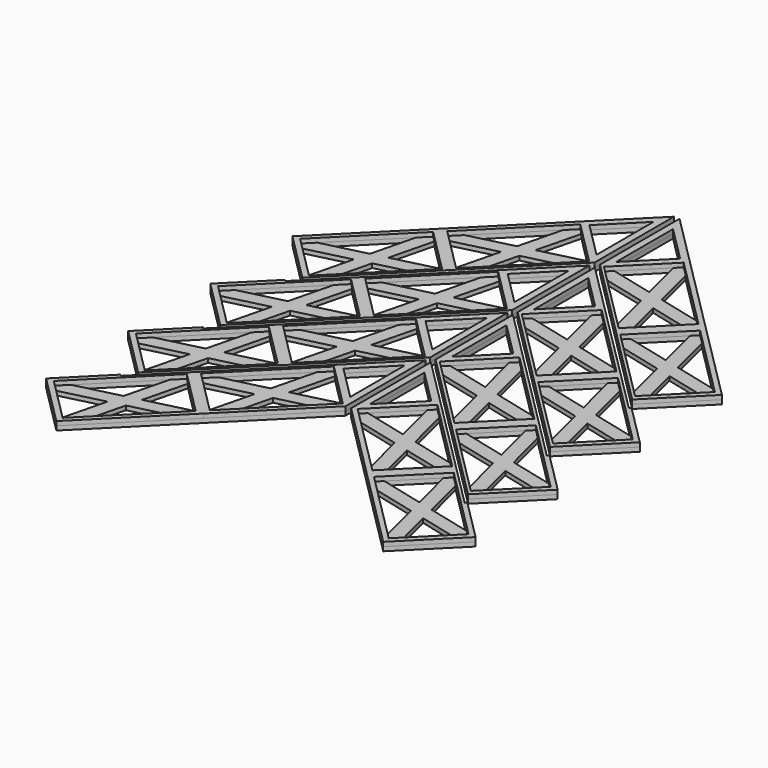
from build123d import *

# Parameters (mm, degrees)
F1_DEPTH = 3
F3_DEPTH = 3
F5_DEPTH = 6
F7_DEPTH = 6


# Not quite as in the source:
# - a feature names something its author has since deleted; it is built from what else it names


with BuildPart() as f1:
    # F0 (on Top) → F1 (new body)
    with BuildSketch(Plane.XY):
        Polygon((-2, -61.6396103068), (-2, -2), (-31.8198051534, -31.8198051534), align=None)
        Polygon((-2, -61.6396103068), (-31.8198051534, -31.8198051534), (-36.8198067184, -36.8198067184), (-2, -71.6396104532), align=None)
        Polygon((-2, -71.6396104532), (-36.8198067184, -36.8198067184), (-95.4594154602, -95.4594154602), (-59.7206892891, -131.1346304254), (-2, -73.3111832249), align=None)
        Polygon((-90.1561136766, -95.1561166906), (-37.1231070285, -42.1231061606), (-5.3033007106, -73.9429101495), (-58.3363073586, -126.9759206794), align=None, mode=Mode.SUBTRACT)
        Polygon((-59.7206892891, -131.1346304254), (-95.4594154602, -95.4594154602), (-154.0990202856, -154.0990288702), (-118.3398738044, -189.8581724084), align=None)
        Polygon((-148.7957204896, -153.795727796), (-95.7627138416, -100.762717266), (-63.9429075236, -132.5825212548), (-116.9759141717, -185.6155317848), align=None, mode=Mode.SUBTRACT)
    extrude(amount=F1_DEPTH)


with BuildPart() as f1b:
    # F0 (on Top) → F1, piece 2 (new body)
    with BuildSketch(Plane.XY):
        Polygon((-123.2896154271, -346.3297840758), (-124.3502800956, -345.2691194021), (-154.0990289767, -375.0178411307), (-117.2792322747, -411.8376540035), (-58.6396110618, -353.198051557), (-94.398746738, -317.4389106458), align=None)
        Polygon((-148.7957294692, -374.7145407415), (-95.7627092344, -321.6815437982), (-63.9429110685, -353.501355939), (-116.9759313032, -406.5343528823), align=None, mode=Mode.SUBTRACT)
        Polygon((-2, -292.5584394851), (-2, -282.558438898), (-30.7591427167, -253.7992961813), (-35.7591450711, -258.7992993562), align=None)
        Polygon((-2, -282.558438898), (-2, -225.0401487453), (-30.7591427167, -253.7992961813), align=None)
        Polygon((-2, -296.5584389525), (-2, -292.5584394851), (-35.7591450711, -258.7992993562), (-94.398746738, -317.4389106458), (-58.6396110618, -353.198051557), align=None)
        Polygon((-90.1561133859, -316.0749487705), (-37.1231086789, -263.0419362996), (-5.3033011963, -294.8617391239), (-58.3363059034, -347.8947515948), align=None, mode=Mode.SUBTRACT)
    extrude(amount=F1_DEPTH)


with BuildPart() as f1c:
    # F0 (on Top) → F1, piece 3 (new body)
    with BuildSketch(Plane.XY):
        Polygon((-123.2896235896, -272.6901718374), (-124.3502835323, -271.62951205), (-154.0990146791, -301.3782501328), (-118.3398697839, -337.1373952008), (-59.7002649834, -278.4977817547), (-94.3987529307, -243.7992988871), align=None)
        Polygon((-116.9759095702, -332.8947529571), (-148.7957170528, -301.0749501328), (-95.7627123456, -248.041937662), (-63.9429048631, -279.8617404862), align=None, mode=Mode.SUBTRACT)
        Polygon((-2, -218.9188283053), (-2, -208.9188285912), (-30.7591438411, -180.1596847501), (-35.7591485237, -185.1596898292), align=None)
        Polygon((-2, -208.9188285912), (-2, -151.400538628), (-30.7591438411, -180.1596847501), align=None)
        Polygon((-2, -220.7975082642), (-2, -218.9188283053), (-35.7591485237, -185.1596898292), (-94.3987529307, -243.7992988871), (-59.7002649834, -278.4977817547), align=None)
        Polygon((-90.1561143554, -242.435338851), (-37.1231096484, -189.4023263801), (-5.3033021659, -221.2221292043), (-58.336306873, -274.2551416752), align=None, mode=Mode.SUBTRACT)
    extrude(amount=F1_DEPTH)


with BuildPart() as f1d:
    # F0 (on Top) → F1, piece 4 (new body)
    with BuildSketch(Plane.XY):
        Polygon((-2, -135.3278050504), (-2, -77.9680376814), (-30.6798418058, -106.5989096283), align=None)
        Polygon((-2, -145.3363573492), (-2, -135.3278050504), (-30.6798418058, -106.5989096283), (-35.6841106479, -111.5946338508), align=None)
        Polygon((-123.2896209509, -199.050560711), (-124.3502811379, -197.9899006113), (-154.099019893, -227.7386418146), (-118.3398762823, -263.4977828078), (-59.7002682444, -204.8581704429), (-94.374065836, -170.1843779274), align=None)
        Polygon((-95.7627149147, -174.4023288289), (-63.9429093731, -206.2221297122), (-116.9759140802, -259.2551421831), (-148.7957196218, -227.4353412998), align=None, mode=Mode.SUBTRACT)
        Polygon((-2, -147.1578979409), (-2, -145.3363573492), (-35.6841106479, -111.5946338508), (-94.374065836, -170.1843779274), (-59.7002682444, -204.8581704429), align=None)
        Polygon((-37.1231038315, -115.7627173353), (-5.3033006191, -147.5825205477), (-58.336309208, -200.6155291367), (-90.1561124205, -168.7957259243), align=None, mode=Mode.SUBTRACT)
    extrude(amount=F1_DEPTH)


with BuildPart() as f1e:
    # F0 (on Top) → F1, piece 5 (new body)
    with BuildSketch(Plane.XY):
        Polygon((31.8198051534, -31.8198051534), (2, -2), (2, -61.6396103068), align=None)
        Polygon((31.8198051534, -31.8198051534), (2, -61.6396103068), (2, -71.6396104532), (36.8198067184, -36.8198067184), align=None)
        Polygon((36.8198067184, -36.8198067184), (2, -71.6396104532), (2, -73.3111832249), (59.7206892891, -131.1346304254), (95.4594154602, -95.4594154602), align=None)
        Polygon((37.1231070285, -42.1231061606), (90.1561136766, -95.1561166906), (58.3363073586, -126.9759206794), (5.3033007106, -73.9429101495), align=None, mode=Mode.SUBTRACT)
        Polygon((154.0990202856, -154.0990288702), (95.4594154602, -95.4594154602), (59.7206892891, -131.1346304254), (118.3398738044, -189.8581724084), align=None)
        Polygon((63.9429075236, -132.5825212548), (95.7627138416, -100.762717266), (148.7957204896, -153.795727796), (116.9759141717, -185.6155317848), align=None, mode=Mode.SUBTRACT)
    extrude(amount=F1_DEPTH)


with BuildPart() as f1f:
    # F0 (on Top) → F1, piece 6 (new body)
    with BuildSketch(Plane.XY):
        Polygon((30.6798418058, -106.5989096283), (2, -77.9680376814), (2, -135.3278050504), align=None)
        Polygon((30.6798418058, -106.5989096283), (2, -135.3278050504), (2, -145.3363573492), (35.6841106479, -111.5946338508), align=None)
        Polygon((35.6841106479, -111.5946338508), (2, -145.3363573492), (2, -147.1578979409), (59.7002682444, -204.8581704429), (94.374065836, -170.1843779274), align=None)
        Polygon((58.336309208, -200.6155291367), (5.3033006191, -147.5825205477), (37.1231038315, -115.7627173353), (90.1561124205, -168.7957259243), align=None, mode=Mode.SUBTRACT)
        Polygon((123.2896209509, -199.050560711), (94.374065836, -170.1843779274), (59.7002682444, -204.8581704429), (118.3398762823, -263.4977828078), (154.099019893, -227.7386418146), (124.3502811379, -197.9899006113), align=None)
        Polygon((63.9429093731, -206.2221297122), (95.7627149147, -174.4023288289), (148.7957196217, -227.4353412998), (116.9759140802, -259.2551421831), align=None, mode=Mode.SUBTRACT)
    extrude(amount=F1_DEPTH)


with BuildPart() as f1g:
    # F0 (on Top) → F1, piece 7 (new body)
    with BuildSketch(Plane.XY):
        Polygon((30.7591438411, -180.1596847501), (2, -151.400538628), (2, -208.9188285912), align=None)
        Polygon((30.7591438411, -180.1596847501), (2, -208.9188285912), (2, -218.9188283053), (35.7591485237, -185.1596898292), align=None)
        Polygon((35.7591485237, -185.1596898292), (2, -218.9188283053), (2, -220.7975082642), (59.7002649834, -278.4977817547), (94.3987529307, -243.7992988871), align=None)
        Polygon((5.3033021659, -221.2221292043), (37.1231096484, -189.4023263801), (90.1561143554, -242.435338851), (58.336306873, -274.2551416752), align=None, mode=Mode.SUBTRACT)
        Polygon((123.2896235896, -272.6901718374), (94.3987529307, -243.7992988871), (59.7002649834, -278.4977817547), (118.3398697839, -337.1373952008), (154.0990146791, -301.3782501328), (124.3502835323, -271.62951205), align=None)
        Polygon((116.9759095702, -332.8947529571), (63.9429048631, -279.8617404862), (95.7627123456, -248.041937662), (148.7957170528, -301.0749501328), align=None, mode=Mode.SUBTRACT)
    extrude(amount=F1_DEPTH)


with BuildPart() as f1h:
    # F0 (on Top) → F1, piece 8 (new body)
    with BuildSketch(Plane.XY):
        Polygon((30.7591427167, -253.7992961813), (2, -225.0401487453), (2, -282.558438898), align=None)
        Polygon((30.7591427167, -253.7992961813), (2, -282.558438898), (2, -292.5584394851), (35.7591450711, -258.7992993562), align=None)
        Polygon((35.7591450711, -258.7992993562), (2, -292.5584394851), (2, -296.5584389525), (58.6396110618, -353.198051557), (94.398746738, -317.4389106458), align=None)
        Polygon((5.3033011963, -294.8617391239), (37.1231086789, -263.0419362996), (90.1561133859, -316.0749487705), (58.3363059034, -347.8947515948), align=None, mode=Mode.SUBTRACT)
        Polygon((123.2896154271, -346.3297840758), (94.398746738, -317.4389106458), (58.6396110618, -353.198051557), (117.2792322747, -411.8376540035), (154.0990289767, -375.0178411307), (124.3502800956, -345.2691194021), align=None)
        Polygon((95.7627092344, -321.6815437982), (148.7957294692, -374.7145407415), (116.9759313032, -406.5343528823), (63.9429110685, -353.501355939), align=None, mode=Mode.SUBTRACT)
    extrude(amount=F1_DEPTH)


with BuildPart() as f3:
    # F2 (on face) → F3 (new body)
    with BuildSketch(Plane(origin=(0, 0, 0), x_dir=(1, 0, 0), z_dir=(0, 0, -1))):
        Polygon((2, 73.3111832249), (2, 2), (154.0990202856, 154.0990288702), (118.3398738044, 189.8581724084), align=None)
        Polygon((33.000001252, 46.2462116354), (9.4264064871, 69.8198046747), (40.8578647357, 77.6776704592), align=None, mode=Mode.SUBTRACT)
        Polygon((12.1751431684, 80.8147531103), (51.4644649007, 120.1040777185), (43.606601417, 88.6726188947), align=None, mode=Mode.SUBTRACT)
        Polygon((83.2842712187, 88.2842737297), (43.9949494864, 48.9949491215), (51.8528129701, 80.4264079453), align=None, mode=Mode.SUBTRACT)
        Polygon((62.4594131351, 122.8528152047), (86.0330079, 99.2792221653), (54.6015496514, 91.4213563809), align=None, mode=Mode.SUBTRACT)
        Polygon((91.6396080651, 104.8858227407), (68.0660133001, 128.4594157801), (99.4974715488, 136.3172815645), align=None, mode=Mode.SUBTRACT)
        Polygon((141.9238780318, 146.9238848351), (102.6345562995, 107.6345602269), (110.4924197831, 139.0660190507), align=None, mode=Mode.SUBTRACT)
        Polygon((70.8147499815, 139.4543642157), (110.1040717138, 178.7436888239), (102.2462082301, 147.3122300001), align=None, mode=Mode.SUBTRACT)
        Polygon((121.0990199482, 181.4924263101), (144.6726147131, 157.9188332707), (113.2411564645, 150.0609674863), align=None, mode=Mode.SUBTRACT)
    extrude(amount=F3_DEPTH)


with BuildPart() as f3b:
    # F2 (on face) → F3, piece 2 (new body)
    with BuildSketch(Plane(origin=(0, 0, 0), x_dir=(1, 0, 0), z_dir=(0, 0, -1))):
        Polygon((2, 147.1578979409), (2, 77.9680376814), (123.2896209509, 199.050560711), (124.3502811379, 197.9899006113), (154.099019893, 227.7386418146), (118.3398762823, 263.4977828078), align=None)
        Polygon((32.9999982725, 119.8858228944), (9.4264061781, 143.4594149887), (40.8578635022, 151.3172802184), align=None, mode=Mode.SUBTRACT)
        Polygon((83.2842694029, 161.9238829067), (43.9949468491, 122.6345603529), (51.8528120788, 154.066017677), align=None, mode=Mode.SUBTRACT)
        Polygon((12.1751436366, 154.4543635653), (51.4644661905, 193.7436861192), (43.6066009607, 162.3122287951), align=None, mode=Mode.SUBTRACT)
        Polygon((62.4594147671, 196.4924235777), (86.0330068614, 172.9188314833), (54.6015495373, 165.0609662536), align=None, mode=Mode.SUBTRACT)
        Polygon((91.6396090538, 178.5254340861), (68.0660152339, 202.0990244549), (99.4974719828, 209.9568919854), align=None, mode=Mode.SUBTRACT)
        Polygon((141.9238771072, 220.5634977792), (102.6345574293, 181.2741723495), (110.4924203583, 212.7056302487), align=None, mode=Mode.SUBTRACT)
        Polygon((70.8147518877, 213.0939732327), (110.1040715656, 252.3832986625), (102.2462086366, 220.9518407632), align=None, mode=Mode.SUBTRACT)
        Polygon((121.099019941, 255.1320369258), (144.6726137609, 231.558446557), (113.241157012, 223.7005790266), align=None, mode=Mode.SUBTRACT)
    extrude(amount=F3_DEPTH)


with BuildPart() as f3c:
    # F2 (on face) → F3, piece 3 (new body)
    with BuildSketch(Plane(origin=(0, 0, 0), x_dir=(1, 0, 0), z_dir=(0, 0, -1))):
        Polygon((154.0990146791, 301.3782501328), (118.3398697839, 337.1373952008), (2, 220.7975082642), (2, 151.400538628), (123.2896235896, 272.6901718374), (124.3502835323, 271.62951205), align=None)
        Polygon((40.8578660543, 224.9568908153), (33.000003721, 193.5254317039), (9.4264080933, 217.0990238805), align=None, mode=Mode.SUBTRACT)
        Polygon((43.6066023333, 235.9518393515), (12.1751443722, 228.0939724167), (51.4644646666, 267.3832984629), align=None, mode=Mode.SUBTRACT)
        Polygon((51.8528141881, 227.7056287039), (83.2842721491, 235.5634956387), (43.9949518547, 196.2741695924), align=None, mode=Mode.SUBTRACT)
        Polygon((54.601550467, 238.7005772401), (62.4594128004, 270.1320363514), (86.033008428, 246.5584441749), align=None, mode=Mode.SUBTRACT)
        Polygon((99.4974687516, 283.5965020972), (91.6396064182, 252.1650429858), (68.0660107905, 275.7386351624), align=None, mode=Mode.SUBTRACT)
        Polygon((102.2462050305, 294.5914506333), (70.8147470695, 286.7335836986), (110.1040673639, 326.0229097447), align=None, mode=Mode.SUBTRACT)
        Polygon((110.4924168853, 286.3452399857), (141.9238748464, 294.2031069205), (102.634554552, 254.9137808744), align=None, mode=Mode.SUBTRACT)
        Polygon((113.2411531643, 297.3401885218), (121.0990154976, 328.7716476333), (144.6726111254, 305.1980554566), align=None, mode=Mode.SUBTRACT)
    extrude(amount=F3_DEPTH)


with BuildPart() as f3d:
    # F2 (on face) → F3, piece 4 (new body)
    with BuildSketch(Plane(origin=(0, 0, 0), x_dir=(1, 0, 0), z_dir=(0, 0, -1))):
        Polygon((2, 296.5584389525), (2, 225.0401487453), (123.2896154271, 346.3297840758), (124.3502800956, 345.2691194021), (154.0990289767, 375.0178411307), (117.2792322747, 411.8376540035), align=None)
        Polygon((33.0000027514, 267.1650416234), (9.4264071237, 290.7386338), (40.8578649974, 298.5965006474), align=None, mode=Mode.SUBTRACT)
        Polygon((83.2842709742, 309.2031053528), (43.9949506799, 269.9137793066), (51.8528131006, 301.3452385054), align=None, mode=Mode.SUBTRACT)
        Polygon((12.1751433489, 301.7335823953), (51.4644634917, 341.022908177), (43.6066012804, 309.5914492918), align=None, mode=Mode.SUBTRACT)
        Polygon((62.4594118308, 343.7716462709), (86.0330074585, 320.1980540943), (54.6015494358, 312.340187175), align=None, mode=Mode.SUBTRACT)
        Polygon((99.4974761378, 357.2361072273), (91.6396045142, 325.8046503292), (68.0660157887, 349.378249408), align=None, mode=Mode.SUBTRACT)
        Polygon((110.4924249682, 359.9848418925), (141.9238854561, 367.8426997465), (102.6345533938, 328.5533850524), align=None, mode=Mode.SUBTRACT)
        Polygon((102.2462157015, 368.2310551291), (70.8147554922, 360.3731973448), (110.1040872902, 399.6625118873), align=None, mode=Mode.SUBTRACT)
        Polygon((113.241164519, 370.979789791), (121.0990360234, 402.4112463513), (144.6726245025, 378.8376475189), align=None, mode=Mode.SUBTRACT)
    extrude(amount=F3_DEPTH)


with BuildPart() as f3e:
    # F2 (on face) → F3, piece 5 (new body)
    with BuildSketch(Plane(origin=(0, 0, 0), x_dir=(1, 0, 0), z_dir=(0, 0, -1))):
        Polygon((-2, 77.9680376814), (-2, 147.1578979409), (-118.3398762823, 263.4977828078), (-154.099019893, 227.7386418146), (-124.3502811379, 197.9899006113), (-123.2896209509, 199.050560711), align=None)
        Polygon((-141.9238771072, 220.5634977792), (-110.4924203583, 212.7056302487), (-102.6345574293, 181.2741723495), align=None, mode=Mode.SUBTRACT)
        Polygon((-99.4974719828, 209.9568919854), (-68.0660152339, 202.0990244549), (-91.6396090538, 178.5254340861), align=None, mode=Mode.SUBTRACT)
        Polygon((-43.9949468491, 122.6345603529), (-83.2842694029, 161.9238829067), (-51.8528120788, 154.066017677), align=None, mode=Mode.SUBTRACT)
        Polygon((-40.8578635022, 151.3172802184), (-9.4264061781, 143.4594149887), (-32.9999982725, 119.8858228944), align=None, mode=Mode.SUBTRACT)
        Polygon((-54.6015495373, 165.0609662536), (-86.0330068614, 172.9188314833), (-62.4594147671, 196.4924235777), align=None, mode=Mode.SUBTRACT)
        Polygon((-12.1751436366, 154.4543635653), (-43.6066009607, 162.3122287951), (-51.4644661905, 193.7436861192), align=None, mode=Mode.SUBTRACT)
        Polygon((-113.241157012, 223.7005790266), (-144.6726137609, 231.558446557), (-121.099019941, 255.1320369258), align=None, mode=Mode.SUBTRACT)
        Polygon((-70.8147518877, 213.0939732327), (-102.2462086366, 220.9518407632), (-110.1040715656, 252.3832986625), align=None, mode=Mode.SUBTRACT)
    extrude(amount=F3_DEPTH)


with BuildPart() as f3f:
    # F2 (on face) → F3, piece 6 (new body)
    with BuildSketch(Plane(origin=(0, 0, 0), x_dir=(1, 0, 0), z_dir=(0, 0, -1))):
        Polygon((-2, 2), (-2, 73.3111832249), (-118.3398738044, 189.8581724084), (-154.0990202856, 154.0990288702), align=None)
        Polygon((-83.2842712187, 88.2842737297), (-51.8528129701, 80.4264079453), (-43.9949494864, 48.9949491215), align=None, mode=Mode.SUBTRACT)
        Polygon((-40.8578647357, 77.6776704592), (-9.4264064871, 69.8198046747), (-33.000001252, 46.2462116354), align=None, mode=Mode.SUBTRACT)
        Polygon((-12.1751431684, 80.8147531103), (-43.606601417, 88.6726188947), (-51.4644649007, 120.1040777185), align=None, mode=Mode.SUBTRACT)
        Polygon((-110.4924197831, 139.0660190507), (-102.6345562995, 107.6345602269), (-141.9238780318, 146.9238848351), align=None, mode=Mode.SUBTRACT)
        Polygon((-99.4974715488, 136.3172815645), (-68.0660133001, 128.4594157801), (-91.6396080651, 104.8858227407), align=None, mode=Mode.SUBTRACT)
        Polygon((-113.2411564645, 150.0609674863), (-144.6726147131, 157.9188332707), (-121.0990199482, 181.4924263101), align=None, mode=Mode.SUBTRACT)
        Polygon((-102.2462082301, 147.3122300001), (-110.1040717138, 178.7436888239), (-70.8147499815, 139.4543642157), align=None, mode=Mode.SUBTRACT)
        Polygon((-54.6015496514, 91.4213563809), (-86.0330079, 99.2792221653), (-62.4594131351, 122.8528152047), align=None, mode=Mode.SUBTRACT)
    extrude(amount=F3_DEPTH)


with BuildPart() as f3g:
    # F2 (on face) → F3, piece 7 (new body)
    with BuildSketch(Plane(origin=(0, 0, 0), x_dir=(1, 0, 0), z_dir=(0, 0, -1))):
        Polygon((-123.2896154271, 346.3297840758), (-2, 225.0401487453), (-2, 296.5584389525), (-117.2792322747, 411.8376540035), (-154.0990289767, 375.0178411307), (-124.3502800956, 345.2691194021), align=None)
        Polygon((-51.8528131006, 301.3452385054), (-43.9949506799, 269.9137793066), (-83.2842709742, 309.2031053528), align=None, mode=Mode.SUBTRACT)
        Polygon((-40.8578649974, 298.5965006474), (-9.4264071237, 290.7386338), (-33.0000027514, 267.1650416234), align=None, mode=Mode.SUBTRACT)
        Polygon((-102.6345533938, 328.5533850524), (-141.9238854561, 367.8426997465), (-110.4924249682, 359.9848418925), align=None, mode=Mode.SUBTRACT)
        Polygon((-68.0660157887, 349.378249408), (-91.6396045142, 325.8046503292), (-99.4974761378, 357.2361072273), align=None, mode=Mode.SUBTRACT)
        Polygon((-144.6726245025, 378.8376475189), (-121.0990360234, 402.4112463513), (-113.241164519, 370.979789791), align=None, mode=Mode.SUBTRACT)
        Polygon((-110.1040872902, 399.6625118873), (-70.8147554922, 360.3731973448), (-102.2462157015, 368.2310551291), align=None, mode=Mode.SUBTRACT)
        Polygon((-54.6015494358, 312.340187175), (-86.0330074585, 320.1980540943), (-62.4594118308, 343.7716462709), align=None, mode=Mode.SUBTRACT)
        Polygon((-12.1751433489, 301.7335823953), (-43.6066012804, 309.5914492918), (-51.4644634917, 341.022908177), align=None, mode=Mode.SUBTRACT)
    extrude(amount=F3_DEPTH)


with BuildPart() as f3h:
    # F2 (on face) → F3, piece 8 (new body)
    with BuildSketch(Plane(origin=(0, 0, 0), x_dir=(1, 0, 0), z_dir=(0, 0, -1))):
        Polygon((-2, 151.400538628), (-2, 220.7975082642), (-118.3398697839, 337.1373952008), (-154.0990146791, 301.3782501328), (-124.3502835323, 271.62951205), (-123.2896235896, 272.6901718374), align=None)
        Polygon((-102.634554552, 254.9137808744), (-141.9238748464, 294.2031069205), (-110.4924168853, 286.3452399857), align=None, mode=Mode.SUBTRACT)
        Polygon((-68.0660107905, 275.7386351624), (-91.6396064182, 252.1650429858), (-99.4974687516, 283.5965020972), align=None, mode=Mode.SUBTRACT)
        Polygon((-110.1040673639, 326.0229097447), (-70.8147470695, 286.7335836986), (-102.2462050305, 294.5914506333), align=None, mode=Mode.SUBTRACT)
        Polygon((-43.9949518547, 196.2741695924), (-83.2842721491, 235.5634956387), (-51.8528141881, 227.7056287039), align=None, mode=Mode.SUBTRACT)
        Polygon((-86.033008428, 246.5584441749), (-62.4594128004, 270.1320363514), (-54.601550467, 238.7005772401), align=None, mode=Mode.SUBTRACT)
        Polygon((-9.4264080933, 217.0990238805), (-33.000003721, 193.5254317039), (-40.8578660543, 224.9568908153), align=None, mode=Mode.SUBTRACT)
        Polygon((-51.4644646666, 267.3832984629), (-12.1751443722, 228.0939724167), (-43.6066023333, 235.9518393515), align=None, mode=Mode.SUBTRACT)
        Polygon((-144.6726111254, 305.1980554566), (-121.0990154976, 328.7716476333), (-113.2411531643, 297.3401885218), align=None, mode=Mode.SUBTRACT)
    extrude(amount=F3_DEPTH)


with BuildPart() as f5_tool:
    # F4 (on face) → F5 (new body)
    with BuildSketch(Plane.XY.offset(3)):
        Polygon((-7, -65.1751442127), (-7, -14.0710678119), (-32.5520382004, -39.6231060123), align=None)
        Polygon((32.5520382004, -39.6231060123), (7, -14.0710678119), (7, -65.1751442127), align=None)
        Polygon((-7, -138.8147543671), (-7, -90.0245339373), (-31.3951102149, -114.4196441522), align=None)
        Polygon((31.3951102149, -114.4196441522), (7, -90.0245339373), (7, -138.8147543671), align=None)
    extrude(amount=-F5_DEPTH)


with BuildPart() as f1_1:
    add(f1.part)

    # F5: cut by f5_tool
    add(f5_tool.part, mode=Mode.SUBTRACT)


with BuildPart() as f1d_1:
    add(f1d.part)

    # F5: cut by f5_tool
    add(f5_tool.part, mode=Mode.SUBTRACT)


with BuildPart() as f1e_1:
    add(f1e.part)

    # F5: cut by f5_tool
    add(f5_tool.part, mode=Mode.SUBTRACT)


with BuildPart() as f1f_1:
    add(f1f.part)

    # F5: cut by f5_tool
    add(f5_tool.part, mode=Mode.SUBTRACT)


with BuildPart() as f3_1:
    add(f3.part)

    # F5: cut by f5_tool
    add(f5_tool.part, mode=Mode.SUBTRACT)


with BuildPart() as f3b_1:
    add(f3b.part)

    # F5: cut by f5_tool
    add(f5_tool.part, mode=Mode.SUBTRACT)


with BuildPart() as f3e_1:
    add(f3e.part)

    # F5: cut by f5_tool
    add(f5_tool.part, mode=Mode.SUBTRACT)


with BuildPart() as f3f_1:
    add(f3f.part)

    # F5: cut by f5_tool
    add(f5_tool.part, mode=Mode.SUBTRACT)


with BuildPart() as f7_tool:
    # F6 (on face) → F7 (new body)
    with BuildSketch(Plane.XY.offset(3)):
        Polygon((-7, -212.461745006), (-7, -163.4716074523), (-31.4950687769, -187.9666798151), align=None)
        Polygon((-7, -237.111218124), (-31.4913773698, -261.6025990792), (-7, -286.0939728636), align=None)
        Polygon((31.4913773698, -261.6025990792), (7, -237.111218124), (7, -286.0939728636), align=None)
        Polygon((31.4950687769, -187.9666798151), (7, -163.4716074523), (7, -212.461745006), align=None)
    extrude(amount=-F7_DEPTH)


with BuildPart() as f1b_1:
    add(f1b.part)

    # F7: cut by f7_tool
    add(f7_tool.part, mode=Mode.SUBTRACT)


with BuildPart() as f1c_1:
    add(f1c.part)

    # F7: cut by f7_tool
    add(f7_tool.part, mode=Mode.SUBTRACT)


with BuildPart() as f1g_1:
    add(f1g.part)

    # F7: cut by f7_tool
    add(f7_tool.part, mode=Mode.SUBTRACT)


with BuildPart() as f1h_1:
    add(f1h.part)

    # F7: cut by f7_tool
    add(f7_tool.part, mode=Mode.SUBTRACT)


with BuildPart() as f3c_1:
    add(f3c.part)

    # F7: cut by f7_tool
    add(f7_tool.part, mode=Mode.SUBTRACT)


with BuildPart() as f3d_1:
    add(f3d.part)

    # F7: cut by f7_tool
    add(f7_tool.part, mode=Mode.SUBTRACT)


with BuildPart() as f3g_1:
    add(f3g.part)

    # F7: cut by f7_tool
    add(f7_tool.part, mode=Mode.SUBTRACT)


with BuildPart() as f3h_1:
    add(f3h.part)

    # F7: cut by f7_tool
    add(f7_tool.part, mode=Mode.SUBTRACT)


solid = Compound([f1_1.part, f1d_1.part, f1e_1.part, f1f_1.part, f3_1.part, f3b_1.part, f3e_1.part, f3f_1.part, f1b_1.part, f1c_1.part, f1g_1.part, f1h_1.part, f3c_1.part, f3d_1.part, f3g_1.part, f3h_1.part])
